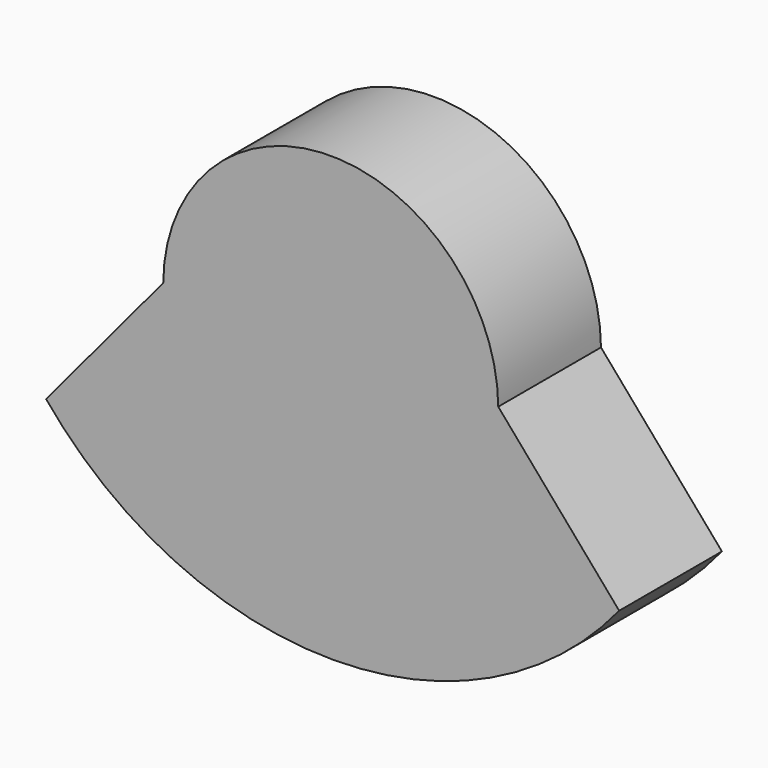
from build123d import *

# Parameters (mm, degrees)
F3_DEPTH = 25.4


# Not quite as in the source:
# - the program builds the solid bodies; features that only make, move or delete a surface that nothing else refers to are left out


with BuildPart() as f3:
    # F2 (on Front) → F3 (new body)
    with BuildSketch(Plane.XZ):
        with BuildLine():
            Line((56.9261387327, -27.7429844416), (33.0086089671, 0))
            ThreePointArc((33.0086089671, 0), (-0.1195967197, 32.9251550814), (-33.2478024065, 0))
            Line((-33.2478024065, 0), (-56.4171377424, -27.7429844416))
            ThreePointArc((-56.4171377424, -27.7429844416), (0.2545004951, -54.6890634565), (56.9261387327, -27.7429844416))
        make_face()
    extrude(amount=F3_DEPTH)


solid = f3.part
